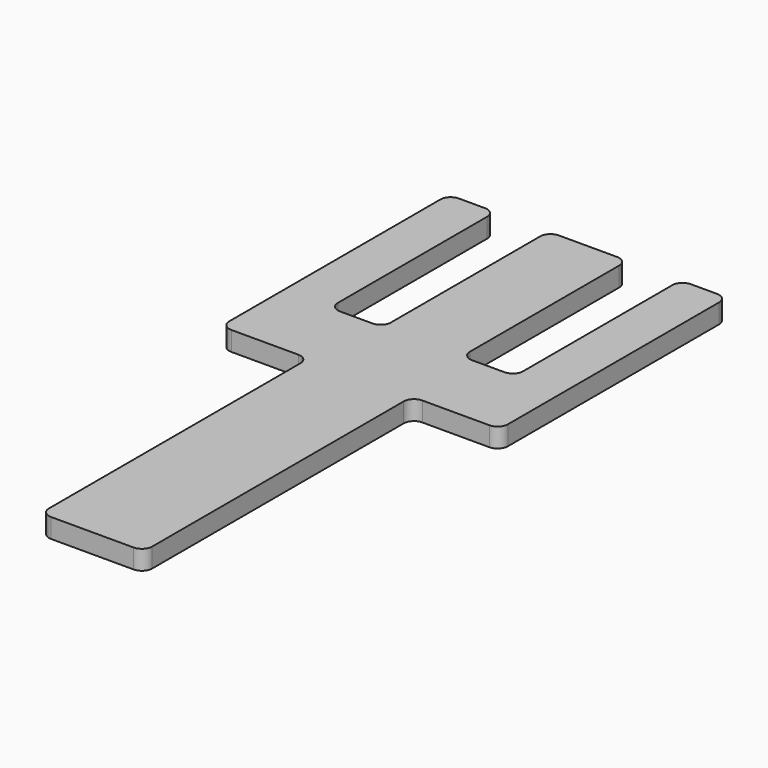
from build123d import *

# Parameters (mm, degrees)
F1_DEPTH = 9.525
F2_R     = 5.08


# Not quite as in the source:
# - a length typed as a fraction of an inch, garbled in the dataset ("3 / 203.2 mm" for 3/8 in), is restored


with BuildPart() as f1:
    # F0 (on Top) → F1 (new body)
    with BuildSketch(Plane.XY):
        Polygon((19.44, 304.8), (0, 304.8), (-19.44, 304.8), (-19.44, 202.9), (-45.56, 202.9), (-45.56, 304.8), (-68.56, 304.8), (-68.56, 164.8), (-25.4, 164.8), (-25.4, 0), (0, 0), (25.4, 0), (25.4, 164.8), (68.56, 164.8), (68.56, 304.8), (45.56, 304.8), (45.56, 202.9), (19.44, 202.9), align=None)
    extrude(amount=F1_DEPTH)

    # F2
    f2_edges = [f1.edges().sort_by_distance(p)[0] for p in [
        (68.56, 304.8, 4.7625),
        (45.56, 304.8, 4.7625),
        (19.44, 304.8, 4.7625),
        (-19.44, 304.8, 4.7625),
        (-45.56, 304.8, 4.7625),
        (-68.56, 304.8, 4.7625),
        (68.56, 164.8, 4.7625),
        (-25.4, 164.8, 4.7625),
        (-68.56, 164.8, 4.7625),
        (-45.56, 202.9, 4.7625),
        (19.44, 202.9, 4.7625),
        (-19.44, 202.9, 4.7625),
        (45.56, 202.9, 4.7625),
        (25.4, 164.8, 4.7625),
        (25.4, 0, 4.7625),
        (-25.4, 0, 4.7625),
    ]]
    fillet(f2_edges, radius=F2_R)


solid = f1.part
